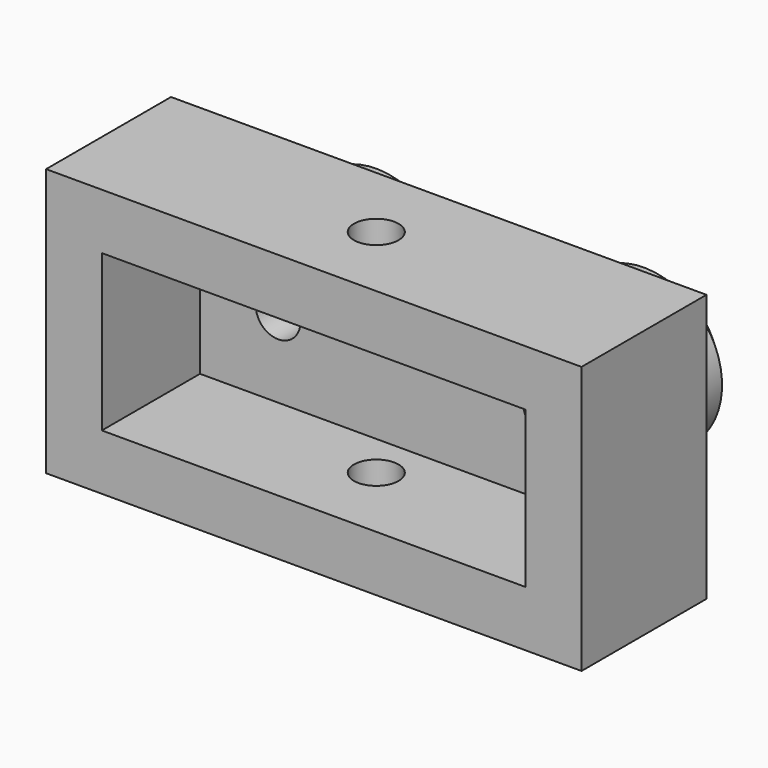
from build123d import *

# Parameters (mm, degrees)
F0_W     = 76.2
F0_H     = 38.1
F1_DEPTH = 25.4
F2_R     = 11.1125
F3_DEPTH = 12.7
F4_SIZE2 = 3.175
F4_SIZE  = 3.175
F5_SIZE2 = 3.175
F5_SIZE  = 3.175
F6_T     = 7.9375
F7_R     = 3.175
F8_DEPTH = 38.1


# Not quite as in the source:
# - a shell that OpenCascade refuses in one call is made with other operations: the cavity is built on its own and cut out


with BuildPart() as f1:
    # F0 (on Front) → F1 (new body)
    with BuildSketch(Plane.XZ):
        Rectangle(F0_W, F0_H)
    extrude(amount=F1_DEPTH)

    # F2 (on face) → F3 (join)
    with BuildSketch(Plane(origin=(0, 0, 0), x_dir=(-1, 0, 0), z_dir=(0, 1, 0))):
        with Locations((-19.05, 0)):
            Circle(F2_R)
        with Locations((19.05, 0)):
            Circle(F2_R)
    extrude(amount=F3_DEPTH)

    # F4
    f4_edges = [f1.edges().sort_by_distance(p)[0] for p in [
        (30.1625, 12.7, 0),
        (-7.9375, 12.7, 0),
    ]]
    chamfer(f4_edges, length=F4_SIZE, length2=F4_SIZE2)

    # F5
    f5_edges = [f1.edges().sort_by_distance(p)[0] for p in [
        (0, 0, 19.05),
        (38.1, 0, 0),
        (0, 0, -19.05),
        (-38.1, 0, 0),
    ]]
    chamfer(f5_edges, length=F5_SIZE, length2=F5_SIZE2)

    # F6: shell of thickness 7.9375, made by hand


with BuildPart() as f6_core1:
    # F6_t2: copy of F1
    add(f1.part)

    # the walls: a layer under each face that stays
    f6_faces = [f6_core1.faces().sort_by_distance(p)[0] for p in [
        (0, 0, 0),
        (0, -1.5875, 17.4625),
        (36.5125, -1.5875, 0),
        (-36.5125, -1.5875, 0),
        (0, -1.5875, -17.4625),
        (-7.9375, 4.7625, 0),
        (30.1625, 4.7625, 0),
        (0, -14.2875, 19.05),
        (38.1, -14.2875, 0),
        (-38.1, -14.2875, 0),
        (0, -14.2875, -19.05),
        (-9.525, 11.1125, 0),
        (28.575, 11.1125, 0),
        (-19.05, 12.7, 0),
        (19.05, 12.7, 0),
    ]]
    thicken(f6_faces, amount=-F6_T, mode=Mode.SUBTRACT)

    # F6_s3 → F6_t4 (revolve, cut)
    with BuildSketch(Plane.XY):
        Polygon((-30.241875, 0.079375), (-30.1625, -7.9375), (-22.225, -7.9375), (-22.225, 0), align=None)
    revolve(axis=Axis((-19.05, 0, 0), (0, 1, 0)), mode=Mode.SUBTRACT)

    # F6_s5 → F6_t6 (revolve, cut)
    with BuildSketch(Plane.XY):
        Polygon((7.858125, 0.079375), (7.9375, -7.9375), (15.875, -7.9375), (15.875, 0), align=None)
    revolve(axis=Axis((19.05, 0, 0), (0, 1, 0)), mode=Mode.SUBTRACT)


with BuildPart() as f1_1:
    add(f1.part)

    # what is left inside the walls is the cavity
    f6_cavity = [f6_core1.part.solids().sort_by_distance(p)[0] for p in [
        (0, -25.320625, -3.704167),
    ]]
    add(f6_cavity, mode=Mode.SUBTRACT)

    # F7 (on face) → F8 (cut)
    with BuildSketch(Plane.XY.offset(19.05)):
        with Locations((0, -14.2875)):
            Circle(F7_R)
    extrude(amount=-F8_DEPTH, mode=Mode.SUBTRACT)


solid = f1_1.part
